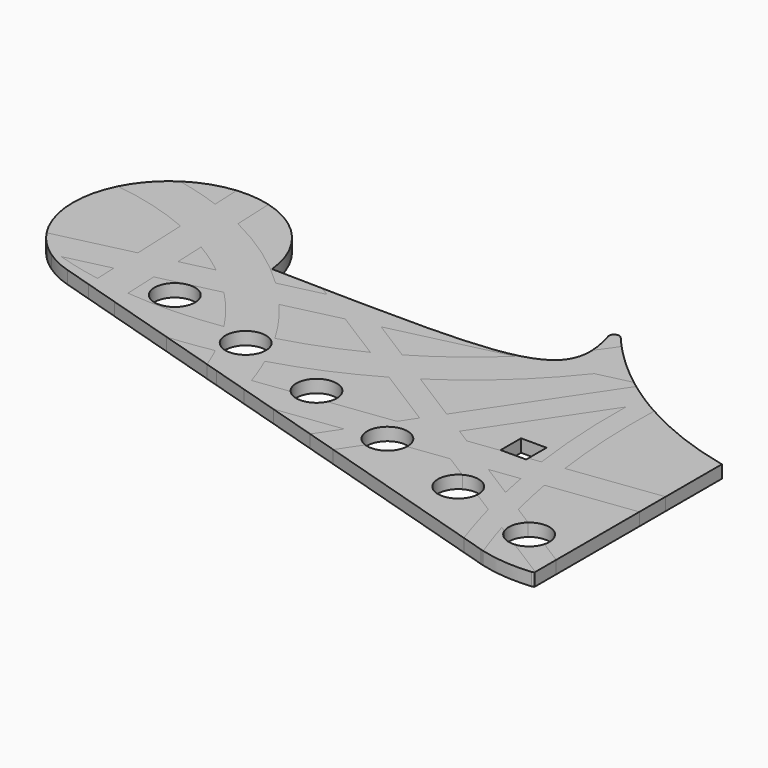
from build123d import *

# Parameters (mm, degrees)
F2_DEPTH    = 3.175
F3_DEPTH    = 3.175
F4_DEPTH    = 3.175
F5_R        = 5.0419
F6_DEPTH    = 3.1760001
F7_T1_DEPTH = 45.676518948
F8_W        = 6.35
F8_H        = 6.35
F9_DEPTH    = 25.4


# Not quite as in the source:
# - a fillet or chamfer that OpenCascade refuses, or shapes differently, is made with other operations: its cross-section is extruded or revolved along the edge and cut away or added
# - a feature names something its author has since deleted; it is built from what else it names


with BuildPart() as f2:
    # F1 (on Top) → F2 (new body)
    with BuildSketch(Plane.XY):
        with BuildLine():
            ThreePointArc((42.4964314187, 15.2975389884), (41.0489158835, 16.1252283316), (39.6171787622, 16.9799210768))
            Line((39.6171787622, 16.9799210768), (37.1046395912, 13.2316301906))
            ThreePointArc((37.1046395912, 13.2316301906), (37.366013418, -0.9466040935), (38.7394922855, -15.0605758765))
            Line((38.7394922855, -15.0605758765), (44.0297445972, -14.3774880883))
            ThreePointArc((44.0297445972, -14.3774880883), (42.6327723421, 0.4274569434), (42.4964314187, 15.2975389884))
        make_face()
        with BuildLine():
            Line((37.1046395912, 13.2316301906), (39.6171787622, 16.9799210768))
            ThreePointArc((39.6171787622, 16.9799210768), (38.4473968067, 17.7056848073), (37.2889933653, 18.4494752905))
            ThreePointArc((37.2889933653, 18.4494752905), (37.1779511751, 15.8412192781), (37.1046395912, 13.2316301906))
        make_face()
        with BuildLine():
            Line((18.2347737019, -14.9190737474), (37.1046395912, 13.2316301906))
            ThreePointArc((37.1046395912, 13.2316301906), (37.1779511751, 15.8412192781), (37.2889933653, 18.4494752905))
            ThreePointArc((37.2889933653, 18.4494752905), (35.2714811063, 19.8067738157), (33.291844794, 21.2187423255))
            Line((33.291844794, 21.2187423255), (11.7897327142, -10.8588354777))
            Line((11.7897327142, -10.8588354777), (18.2347737019, -14.9190737474))
        make_face()
        Polygon((21.909005611, -17.2337614333), (18.2347737019, -14.9190737474), (16.1880374428, -17.9724641003), align=None)
        Polygon((16.1880374428, -17.9724641003), (18.2347737019, -14.9190737474), (11.7897327142, -10.8588354777), (8.7250037822, -15.4309017191), (13.3425786538, -18.3398753382), align=None)
        with BuildLine():
            ThreePointArc((40.0179483598, -23.0484418301), (39.3339699918, -19.0616711332), (38.7394922855, -15.0605758765))
            Line((38.7394922855, -15.0605758765), (21.909005611, -17.2337614333))
            Line((21.909005611, -17.2337614333), (32.6492717175, -23.9998998575))
            Line((32.6492717175, -23.9998998575), (40.0179483598, -23.04844183))
        make_face()
        with BuildLine():
            Line((44.0297445972, -14.3774880883), (38.7394922855, -15.0605758765))
            ThreePointArc((38.7394922855, -15.0605758765), (39.3339699918, -19.0616711332), (40.0179483598, -23.0484418301))
            Line((40.0179483598, -23.04844183), (45.3156103763, -22.3643972862))
            ThreePointArc((45.3156103763, -22.3643972862), (44.6265684594, -18.3783660871), (44.0297445972, -14.3774880883))
        make_face()
        with BuildLine():
            Line((66.0969165157, -11.5281314286), (44.0297445972, -14.3774880883))
            ThreePointArc((44.0297445972, -14.3774880883), (44.6265684594, -18.3783660871), (45.3156103763, -22.3643972862))
            Line((45.3156103763, -22.3643972862), (66.0969165157, -19.6810741461))
            Line((66.0969165157, -19.6810741461), (66.0969165157, -11.5281314286))
        make_face()
        Polygon((21.909005611, -17.2337614333), (16.1880374428, -17.9724641003), (15.1700447699, -19.4911399889), (24.0828447602, -25.1060137624), (32.6492717175, -23.9998998575), align=None)
        Polygon((15.1700447699, -19.4911399889), (16.1880374428, -17.9724641003), (13.3425786538, -18.3398753382), align=None)
        with BuildLine():
            Line((8.7250037822, -15.4309017191), (11.7897327142, -10.8588354777))
            Line((11.7897327142, -10.8588354777), (-1.4386667359, -2.5252261497))
            ThreePointArc((-1.4386667359, -2.5252261497), (-4.0267817378, -4.16929298), (-6.661363794, -5.7378185279))
            Line((-6.661363794, -5.7378185279), (8.7250037822, -15.4309017191))
        make_face()
        with BuildLine():
            Line((45.3156103763, -22.3643972862), (40.0179483598, -23.04844183))
            ThreePointArc((40.0179483598, -23.0484418301), (40.6358918873, -26.2586545513), (41.3118678172, -29.4571505199))
            Line((41.3118678172, -29.4571505199), (47.7543417747, -33.5157716153))
            ThreePointArc((47.7543417747, -33.5157716153), (46.4441248758, -27.9599530039), (45.3156103763, -22.3643972862))
        make_face()
        with BuildLine():
            Line((23.5653367152, 20.3479618092), (31.8543854329, 22.2964799735))
            ThreePointArc((31.8543854329, 22.2964799735), (29.6938437842, 24.004445014), (27.5872449715, 25.7785155417))
            ThreePointArc((27.5872449715, 25.7785155417), (25.6195765344, 23.0311809725), (23.5653367152, 20.3479618092))
        make_face()
        Polygon((66.7319165157, -11.4461389791), (66.0969165157, -11.5281314286), (66.0969165157, -19.6810741461), (66.7319165157, -19.5990816966), align=None)
        Polygon((24.0828447602, -25.1060137624), (15.1700447699, -19.4911399889), (10.2051564991, -26.8979281778), align=None)
        Polygon((10.2051564991, -26.8979281778), (15.1700447699, -19.4911399889), (13.3425786538, -18.3398753382), (6.1527769462, -19.2682366821), (0.1698960025, -28.1937007596), align=None)
        Polygon((6.1527769462, -19.2682366821), (13.3425786538, -18.3398753382), (8.7250037822, -15.4309017191), align=None)
        with BuildLine():
            ThreePointArc((-6.661363794, -5.7378185279), (-4.0267817378, -4.16929298), (-1.4386667359, -2.5252261497))
            Line((-1.4386667359, -2.5252261497), (-10.5116171088, 3.1905389469))
            ThreePointArc((-10.5116171088, 3.1905389469), (-13.2464904723, 1.6325505109), (-16.0307927047, 0.16472172))
            Line((-16.0307927047, 0.16472172), (-6.661363794, -5.7378185279))
        make_face()
        with BuildLine():
            Line((-10.5116171088, 3.1905389469), (-1.4386667359, -2.5252261497))
            ThreePointArc((-1.4386667359, -2.5252261497), (11.983278832, 7.905724058), (23.5653367152, 20.3479618092))
            Line((23.5653367152, 20.3479618092), (6.9924854196, 16.4521586978))
            ThreePointArc((6.9924854196, 16.4521586978), (-1.3805057538, 9.3210248182), (-10.5116171088, 3.1905389469))
        make_face()
        with BuildLine():
            Line((41.3118678172, -29.4571505199), (32.6492717175, -23.9998998575))
            Line((32.6492717175, -23.9998998575), (24.0828447602, -25.1060137624))
            Line((24.0828447602, -25.1060137624), (43.1859281666, -37.140548603))
            ThreePointArc((43.1859281666, -37.140548603), (42.2068160775, -33.3091137761), (41.3118678172, -29.4571505199))
        make_face()
        with BuildLine():
            Line((47.7543417747, -33.5157716153), (41.3118678172, -29.4571505199))
            ThreePointArc((41.3118678172, -29.4571505199), (42.2068160775, -33.3091137761), (43.1859281666, -37.140548603))
            Line((43.1859281666, -37.140548603), (49.9469070818, -41.3998210243))
            ThreePointArc((49.9469070818, -41.3998210243), (48.8045830594, -37.4706004897), (47.7543417747, -33.5157716153))
        make_face()
        with BuildLine():
            Line((6.9924854196, 16.4521586978), (23.5653367152, 20.3479618092))
            ThreePointArc((23.5653367152, 20.3479618092), (25.6195765344, 23.0311809725), (27.5872449715, 25.7785155417))
            ThreePointArc((27.5872449715, 25.7785155417), (26.020865796, 27.172423594), (24.4877966317, 28.6028858679))
            Line((24.4877966317, 28.6028858679), (17.1245144057, 26.8719889151))
            add(Edge.make_bspline(
                [(7.6808851652, 17.1163986448), (14.1067211356, 18.8048631178), (17.0282926135, 21.7855138574), (17.1245144057, 26.8719889151)],
                knots=[0.4777006236, 0.4777006236, 0.4777006236, 0.4777006236, 0.7763446793, 0.7763446793, 0.7763446793, 0.7763446793], degree=3))
            ThreePointArc((7.6808851652, 17.1163986448), (7.3375096508, 16.7834243292), (6.9924854196, 16.4521586978))
        make_face()
        with BuildLine():
            Line((66.0969165157, -45.0712022279), (47.7543417747, -33.5157716153))
            ThreePointArc((47.7543417747, -33.5157716153), (48.8045830594, -37.4706004897), (49.9469070818, -41.3998210243))
            Line((49.9469070818, -41.3998210243), (66.0969165157, -51.5739822879))
            Line((66.0969165157, -51.5739822879), (66.0969165157, -45.0712022279))
        make_face()
        with BuildLine():
            Line((17.1245144057, 26.8719889151), (24.4877966317, 28.6028858679))
            ThreePointArc((24.4877966317, 28.6028858679), (22.4906185602, 30.5721371514), (20.5565558022, 32.6034106718))
            ThreePointArc((20.5565558022, 32.6034106718), (18.8719024579, 30.1633774038), (17.1129665679, 27.7763366052))
            add(Edge.make_bspline(
                [(17.1245144057, 26.8719889151), (17.1300825818, 27.1663337688), (17.1261894483, 27.4677304421), (17.1129665679, 27.7763366052)],
                knots=[0.7763446793, 0.7763446793, 0.7763446793, 0.7763446793, 0.7936266555, 0.7936266555, 0.7936266555, 0.7936266555], degree=3))
        make_face()
        Polygon((3.9051852235, -36.2964383336), (10.2051564991, -26.8979281778), (0.1698960025, -28.1937007596), (-3.7024240646, -33.9705587617), align=None)
        with BuildLine():
            Line((0.1698960025, -28.1937007596), (6.1527769462, -19.2682366821))
            Line((6.1527769462, -19.2682366821), (-26.6654353374, -23.5057888287))
            ThreePointArc((-26.6654353374, -23.5057888287), (-26.0722508431, -25.3958668205), (-25.5232745108, -27.2992552847))
            Line((-25.5232745108, -27.2992552847), (-15.8372389855, -30.2605735265))
            Line((-15.8372389855, -30.2605735265), (0.1698960025, -28.1937007596))
        make_face()
        with BuildLine():
            ThreePointArc((-29.6968030266, -15.588280186), (-17.887048807, -11.3459762685), (-6.661363794, -5.7378185279))
            Line((-6.661363794, -5.7378185279), (-16.0307927047, 0.16472172))
            ThreePointArc((-16.0307927047, 0.16472172), (-24.9308801058, -3.7912137914), (-34.1848701937, -6.8284245133))
            ThreePointArc((-34.1848701937, -6.8284245133), (-31.813933797, -11.1433343436), (-29.6968030266, -15.588280186))
        make_face()
        with BuildLine():
            ThreePointArc((-16.0307927047, 0.16472172), (-13.2464904723, 1.6325505109), (-10.5116171088, 3.1905389469))
            Line((-10.5116171088, 3.1905389469), (-21.0854633248, 9.8518363918))
            Line((-21.0854633248, 9.8518363918), (-28.6026932396, 8.0847507426))
            Line((-28.6026932396, 8.0847507426), (-16.0307927047, 0.16472172))
        make_face()
        with BuildLine():
            Line((49.9469070818, -41.3998210243), (43.1859281666, -37.140548603))
            ThreePointArc((43.1859281666, -37.140548603), (44.9597148144, -43.3326667725), (46.9532808608, -49.4575619483))
            Line((46.9532808608, -49.4575619483), (52.654517861, -51.2006050215))
            add(Edge.make_bspline(
                [(52.654517861, -51.2006050215), (52.8721432701, -51.2671397861), (53.0908731316, -51.3311050786), (53.3106253892, -51.392535085)],
                knots=[0, 0, 0, 0, 0.0179188265, 0.0179188265, 0.0179188265, 0.0179188265], degree=3))
            ThreePointArc((53.3106253892, -51.392535085), (51.5535715097, -46.4214898843), (49.9469070818, -41.3998210243))
        make_face()
        with BuildLine():
            Line((-21.0854633248, 9.8518363918), (6.9924854196, 16.4521586978))
            ThreePointArc((6.9924854196, 16.4521586978), (7.3375096508, 16.7834243292), (7.6808851652, 17.1163986448))
            add(Edge.make_bspline(
                [(-29.5465874229, 15.1821639931), (-11.7884739785, 14.9407807553), (0.2741126095, 15.1701814713), (7.6808851652, 17.1163986448)],
                knots=[0.1334670318, 0.1334670318, 0.1334670318, 0.1334670318, 0.4777006236, 0.4777006236, 0.4777006236, 0.4777006236], degree=3))
            Line((-29.5465874229, 15.1821639931), (-21.0854633248, 9.8518363918))
        make_face()
        Polygon((66.7319165157, -45.4712386755), (66.0969165157, -45.0712022279), (66.0969165157, -51.5739822879), (66.7319165157, -51.9740187355), (66.7319165157, -50.6766184161), align=None)
        with BuildLine():
            ThreePointArc((-25.5232745108, -27.2992552847), (-26.0722508431, -25.3958668205), (-26.6654353374, -23.5057888287))
            Line((-26.6654353374, -23.5057888287), (-34.5859869423, -24.5285060372))
            Line((-34.5859869423, -24.5285060372), (-25.5232745108, -27.2992552847))
        make_face()
        with BuildLine():
            Line((-34.5859869423, -24.5285060372), (-26.6654353374, -23.5057888287))
            ThreePointArc((-26.6654353374, -23.5057888287), (-28.082343762, -19.5092164726), (-29.6968030266, -15.588280186))
            ThreePointArc((-29.6968030266, -15.588280186), (-34.8240491393, -16.9555811432), (-40.0132953676, -18.0645843849))
            ThreePointArc((-40.0132953676, -18.0645843849), (-38.7883325091, -20.8009357195), (-37.6743280791, -23.5843053969))
            Line((-37.6743280791, -23.5843053969), (-34.5859869423, -24.5285060372))
        make_face()
        with BuildLine():
            ThreePointArc((-40.0132953676, -18.0645843849), (-34.8240491393, -16.9555811432), (-29.6968030266, -15.588280186))
            ThreePointArc((-29.6968030266, -15.588280186), (-31.813933797, -11.1433343436), (-34.1848701937, -6.8284245133))
            ThreePointArc((-34.1848701937, -6.8284245133), (-39.5644417055, -8.1325608515), (-45.0100273339, -9.1256159374))
            ThreePointArc((-45.0100273339, -9.1256159374), (-42.3580614142, -13.5092403981), (-40.0132953676, -18.0645843849))
        make_face()
        with BuildLine():
            Line((-28.6026932396, 8.0847507426), (-21.0854633248, 9.8518363918))
            Line((-21.0854633248, 9.8518363918), (-29.5465874229, 15.1821639931))
            add(Edge.make_bspline(
                [(-32.4245408212, 15.2244238657), (-31.4490517341, 15.209133599), (-30.4897858638, 15.1949847409), (-29.5465874229, 15.1821639931)],
                knots=[0.1151835251, 0.1151835251, 0.1151835251, 0.1151835251, 0.1334670318, 0.1334670318, 0.1334670318, 0.1334670318], degree=3))
            Line((-32.4245408212, 15.2244238657), (-37.8947338501, 13.9385380129))
            Line((-37.8947338501, 13.9385380129), (-28.6026932396, 8.0847507426))
        make_face()
        with BuildLine():
            Line((-42.4321868943, 4.8338325121), (-28.6026932396, 8.0847507426))
            Line((-28.6026932396, 8.0847507426), (-37.8947338501, 13.9385380129))
            Line((-37.8947338501, 13.9385380129), (-48.6032420976, 11.4212741454))
            ThreePointArc((-48.6032420976, 11.4212741454), (-45.430208748, 8.2095279148), (-42.4321868943, 4.8338325121))
        make_face()
        with BuildLine():
            ThreePointArc((-45.0100273339, -9.1256159374), (-39.5644417055, -8.1325608515), (-34.1848701937, -6.8284245133))
            ThreePointArc((-34.1848701937, -6.8284245133), (-38.0631186166, -0.8237469707), (-42.4321868943, 4.8338325121))
            Line((-42.4321868943, 4.8338325121), (-54.0070813026, 2.1129060495))
            ThreePointArc((-54.0070813026, 2.1129060495), (-49.23676466, -3.2887723983), (-45.0100273339, -9.1256159374))
        make_face()
        with BuildLine():
            ThreePointArc((-50.9314824477, -19.5311865576), (-45.4533242171, -18.9398134331), (-40.0132953676, -18.0645843849))
            ThreePointArc((-40.0132953676, -18.0645843849), (-42.3580614142, -13.5092403981), (-45.0100273339, -9.1256159374))
            ThreePointArc((-45.0100273339, -9.1256159374), (-56.6586871971, -10.1875434452), (-68.3501889524, -9.8301174407))
            Line((-68.3501889524, -9.8301174407), (-68.1593155628, -14.2641093992))
            Line((-68.1593155628, -14.2641093992), (-50.9314824477, -19.5311865576))
        make_face()
        with BuildLine():
            Line((-40.1503334653, 15.3595176307), (-37.8947338501, 13.9385380129))
            Line((-37.8947338501, 13.9385380129), (-32.4245408212, 15.2244238657))
            add(Edge.make_bspline(
                [(-40.1503334653, 15.3595176307), (-37.4693381201, 15.3091877057), (-34.8949173044, 15.2631456884), (-32.4245408212, 15.2244238657)],
                knots=[0.0688814745, 0.0688814745, 0.0688814745, 0.0688814745, 0.1151835251, 0.1151835251, 0.1151835251, 0.1151835251], degree=3))
        make_face()
        with BuildLine():
            Line((-54.0070813026, 2.1129060495), (-42.4321868943, 4.8338325121))
            ThreePointArc((-42.4321868943, 4.8338325121), (-45.430208748, 8.2095279148), (-48.6032420976, 11.4212741454))
            Line((-48.6032420976, 11.4212741454), (-61.0611600505, 8.492774115))
            ThreePointArc((-61.0611600505, 8.492774115), (-57.4323204183, 5.4153983721), (-54.0070813026, 2.1129060495))
        make_face()
        with BuildLine():
            Line((-61.0611600505, 8.492774115), (-48.6032420976, 11.4212741454))
            ThreePointArc((-48.6032420976, 11.4212741454), (-58.6808959079, 19.7062783812), (-69.9077254027, 26.3514797328))
            Line((-69.9077254027, 26.3514797328), (-69.3860241765, 14.2323517303))
            ThreePointArc((-69.3860241765, 14.2323517303), (-65.1262135584, 11.5038038457), (-61.0611600505, 8.492774115))
        make_face()
        with BuildLine():
            Line((-68.7154707451, -1.3446154313), (-54.0070813026, 2.1129060495))
            ThreePointArc((-54.0070813026, 2.1129060495), (-57.4323204183, 5.4153983721), (-61.0611600505, 8.492774115))
            Line((-61.0611600505, 8.492774115), (-69.0580256175, 6.6129398486))
            Line((-69.0580256175, 6.6129398486), (-68.7154707451, -1.3446154313))
        make_face()
        with BuildLine():
            ThreePointArc((-76.8586239766, -8.6668452954), (-72.6173728923, -9.3433207475), (-68.3501889524, -9.8301174407))
            Line((-68.3501889524, -9.8301174407), (-68.7154707451, -1.3446154313))
            Line((-68.7154707451, -1.3446154313), (-77.0890943511, -3.3130147318))
            Line((-77.0890943511, -3.3130147318), (-76.8586239766, -8.6668452954))
        make_face()
        with BuildLine():
            Line((-68.1593155628, -14.2641093992), (-68.3501889524, -9.8301174407))
            ThreePointArc((-68.3501889524, -9.8301174407), (-72.6173728923, -9.3433207475), (-76.8586239766, -8.6668452954))
            Line((-76.8586239766, -8.6668452954), (-76.730479586, -11.6436415815))
            Line((-76.730479586, -11.6436415815), (-68.1593155628, -14.2641093992))
        make_face()
        with BuildLine():
            ThreePointArc((-78.5240021741, 30.0199174278), (-74.1653042963, 28.3044506523), (-69.9077254027, 26.3514797328))
            Line((-69.9077254027, 26.3514797328), (-70.3394310892, 36.3800098813))
            ThreePointArc((-70.3394310892, 36.3800098813), (-74.5513100111, 37.131060612), (-78.829611199, 37.1192200675))
            Line((-78.829611199, 37.1192200675), (-78.5240021741, 30.0199174278))
        make_face()
        with BuildLine():
            Line((-69.3860241765, 14.2323517303), (-69.9077254027, 26.3514797328))
            ThreePointArc((-69.9077254027, 26.3514797328), (-74.1653042963, 28.3044506523), (-78.5240021741, 30.0199174278))
            Line((-78.5240021741, 30.0199174278), (-78.0338005415, 18.6325254977))
            ThreePointArc((-78.0338005415, 18.6325254977), (-73.6382831604, 16.5732133478), (-69.3860241765, 14.2323517303))
        make_face()
        Polygon((-77.0890943511, -3.3130147318), (-68.7154707451, -1.3446154313), (-69.0580256175, 6.6129398486), (-77.4316492235, 4.6445405481), align=None)
        with BuildLine():
            Line((-76.730479586, -11.6436415815), (-76.8586239766, -8.6668452954))
            ThreePointArc((-76.8586239766, -8.6668452954), (-82.5281158651, -7.4551998292), (-88.1144721554, -5.904765565))
            Line((-88.1144721554, -5.904765565), (-90.1562794913, -6.3847360439))
            ThreePointArc((-90.1562794913, -6.3847360439), (-87.0051766902, -8.2121096218), (-83.6129915736, -9.5394465014))
            Line((-83.6129915736, -9.5394465014), (-76.730479586, -11.6436415815))
        make_face()
        with BuildLine():
            Line((-77.4316492235, 4.6445405481), (-69.0580256175, 6.6129398486))
            Line((-69.0580256175, 6.6129398486), (-69.3860241765, 14.2323517303))
            ThreePointArc((-69.3860241765, 14.2323517303), (-73.6382831604, 16.5732133478), (-78.0338005415, 18.6325254977))
            Line((-78.0338005415, 18.6325254977), (-77.4316492235, 4.6445405481))
        make_face()
        with BuildLine():
            Line((-78.0338005415, 18.6325254977), (-78.5240021741, 30.0199174278))
            ThreePointArc((-78.5240021741, 30.0199174278), (-84.1174389484, 31.8289833917), (-89.8225422612, 33.2470986199))
            ThreePointArc((-89.8225422612, 33.2470986199), (-94.4940594414, 29.1935052495), (-97.9690847289, 24.0769740779))
            ThreePointArc((-97.9690847289, 24.0769740779), (-87.8119657312, 22.0485346354), (-78.0338005415, 18.6325254977))
        make_face()
        with BuildLine():
            Line((-88.1144721554, -5.904765565), (-77.0890943511, -3.3130147318))
            Line((-77.0890943511, -3.3130147318), (-77.4316492235, 4.6445405481))
            Line((-77.4316492235, 4.6445405481), (-96.5696239893, 0.1457503093))
            ThreePointArc((-96.5696239893, 0.1457503093), (-94.7885596821, -2.218402202), (-92.7289486745, -4.3442925239))
            ThreePointArc((-92.7289486745, -4.3442925239), (-90.4315734951, -5.1536951694), (-88.1144721554, -5.904765565))
        make_face()
        with BuildLine():
            Line((-90.1562794913, -6.3847360439), (-88.1144721554, -5.904765565))
            ThreePointArc((-88.1144721554, -5.904765565), (-90.4315734951, -5.1536951694), (-92.7289486745, -4.3442925239))
            ThreePointArc((-92.7289486745, -4.3442925239), (-91.4776936841, -5.408743986), (-90.1562794913, -6.3847360439))
        make_face()
    extrude(amount=F2_DEPTH)


with BuildPart() as f3:
    # F1 (on Top) → F3 (new body)
    with BuildSketch(Plane.XY):
        with BuildLine():
            Line((66.0969165157, -19.6810741461), (45.3156103763, -22.3643972862))
            ThreePointArc((45.3156103763, -22.3643972862), (46.4441248758, -27.9599530039), (47.7543417747, -33.5157716153))
            Line((47.7543417747, -33.5157716153), (66.0969165157, -45.0712022279))
            Line((66.0969165157, -45.0712022279), (66.0969165157, -19.6810741461))
        make_face()
        Polygon((66.7319165157, -19.5990816966), (66.0969165157, -19.6810741461), (66.0969165157, -45.0712022279), (66.7319165157, -45.4712386755), align=None)
    extrude(amount=F3_DEPTH)


with BuildPart() as f3b:
    # F1 (on Top) → F3, piece 2 (new body)
    with BuildSketch(Plane.XY):
        with BuildLine():
            ThreePointArc((38.7394922855, -15.0605758765), (37.366013418, -0.9466040935), (37.1046395912, 13.2316301906))
            Line((37.1046395912, 13.2316301906), (18.2347737019, -14.9190737474))
            Line((18.2347737019, -14.9190737474), (21.909005611, -17.2337614333))
            Line((21.909005611, -17.2337614333), (38.7394922855, -15.0605758765))
        make_face()
    extrude(amount=F3_DEPTH)


with BuildPart() as f3c:
    # F1 (on Top) → F3, piece 3 (new body)
    with BuildSketch(Plane.XY):
        with BuildLine():
            ThreePointArc((41.3118678172, -29.4571505199), (40.6358918873, -26.2586545513), (40.0179483598, -23.0484418301))
            Line((40.0179483598, -23.04844183), (32.6492717175, -23.9998998575))
            Line((32.6492717175, -23.9998998575), (41.3118678172, -29.4571505199))
        make_face()
    extrude(amount=F3_DEPTH)


with BuildPart() as f3d:
    # F1 (on Top) → F3, piece 4 (new body)
    with BuildSketch(Plane.XY):
        with BuildLine():
            Line((24.0828447602, -25.1060137624), (10.2051564991, -26.8979281778))
            Line((10.2051564991, -26.8979281778), (3.9051852235, -36.2964383336))
            Line((3.9051852235, -36.2964383336), (46.9532808608, -49.4575619483))
            ThreePointArc((46.9532808608, -49.4575619483), (44.9597148144, -43.3326667725), (43.1859281666, -37.140548603))
            Line((43.1859281666, -37.140548603), (24.0828447602, -25.1060137624))
        make_face()
    extrude(amount=F3_DEPTH)


with BuildPart() as f3e:
    # F1 (on Top) → F3, piece 5 (new body)
    with BuildSketch(Plane.XY):
        with BuildLine():
            Line((66.0969165157, -51.5739822879), (49.9469070818, -41.3998210243))
            ThreePointArc((49.9469070818, -41.3998210243), (51.5535715097, -46.4214898843), (53.3106253892, -51.392535085))
            add(Edge.make_bspline(
                [(53.3106253892, -51.392535085), (57.3951470823, -52.5343308356), (61.832880342, -52.8002504688), (66.0969165157, -52.4098137845)],
                knots=[0.0179188265, 0.0179188265, 0.0179188265, 0.0179188265, 0.3509749519, 0.3509749519, 0.3509749519, 0.3509749519], degree=3))
            Line((66.0969165157, -52.4098137845), (66.0969165157, -51.5739822879))
        make_face()
        with BuildLine():
            Line((66.7319165157, -51.9740187355), (66.0969165157, -51.5739822879))
            Line((66.0969165157, -51.5739822879), (66.0969165157, -52.4098137845))
            ThreePointArc((66.0969165157, -52.4098137845), (66.426687168, -52.3406803211), (66.7319165157, -52.1979807617))
            Line((66.7319165157, -52.1979807617), (66.7319165157, -51.9740187355))
        make_face()
    extrude(amount=F3_DEPTH)


with BuildPart() as f3f:
    # F1 (on Top) → F3, piece 6 (new body)
    with BuildSketch(Plane.XY):
        with BuildLine():
            ThreePointArc((66.0969165157, 6.2159453417), (53.9721180988, 9.9133135519), (42.4964314187, 15.2975389884))
            ThreePointArc((42.4964314187, 15.2975389884), (42.6327723421, 0.4274569434), (44.0297445972, -14.3774880883))
            Line((44.0297445972, -14.3774880883), (66.0969165157, -11.5281314286))
            Line((66.0969165157, -11.5281314286), (66.0969165157, 6.2159453417))
        make_face()
        with BuildLine():
            ThreePointArc((66.7319165157, 6.0732997692), (66.4142859791, 6.1440414601), (66.0969165157, 6.2159453417))
            Line((66.0969165157, 6.2159453417), (66.0969165157, -11.5281314286))
            Line((66.0969165157, -11.5281314286), (66.7319165157, -11.4461389791))
            Line((66.7319165157, -11.4461389791), (66.7319165157, 6.0732997692))
        make_face()
    extrude(amount=F3_DEPTH)


with BuildPart() as f4:
    # F1 (on Top) → F4 (new body)
    with BuildSketch(Plane.XY):
        with BuildLine():
            Line((-69.0580256175, 6.6129398486), (-61.0611600505, 8.492774115))
            ThreePointArc((-61.0611600505, 8.492774115), (-65.1262135584, 11.5038038457), (-69.3860241765, 14.2323517303))
            Line((-69.3860241765, 14.2323517303), (-69.0580256175, 6.6129398486))
        make_face()
    extrude(amount=F4_DEPTH)


with BuildPart() as f4b:
    # F1 (on Top) → F4, piece 2 (new body)
    with BuildSketch(Plane.XY):
        with BuildLine():
            Line((-96.5696239893, 0.1457503093), (-77.4316492235, 4.6445405481))
            Line((-77.4316492235, 4.6445405481), (-78.0338005415, 18.6325254977))
            ThreePointArc((-78.0338005415, 18.6325254977), (-87.8119657312, 22.0485346354), (-97.9690847289, 24.0769740779))
            ThreePointArc((-97.9690847289, 24.0769740779), (-100.4863179642, 11.9232391662), (-96.5696239893, 0.1457503093))
        make_face()
    extrude(amount=F4_DEPTH)


with BuildPart() as f4c:
    # F1 (on Top) → F4, piece 3 (new body)
    with BuildSketch(Plane.XY):
        with BuildLine():
            ThreePointArc((-89.8225422612, 33.2470986199), (-84.1174389484, 31.8289833917), (-78.5240021741, 30.0199174278))
            Line((-78.5240021741, 30.0199174278), (-78.829611199, 37.1192200675))
            ThreePointArc((-78.829611199, 37.1192200675), (-84.5656995824, 35.8634472767), (-89.8225422612, 33.2470986199))
        make_face()
    extrude(amount=F4_DEPTH)


with BuildPart() as f4d:
    # F1 (on Top) → F4, piece 4 (new body)
    with BuildSketch(Plane.XY):
        with BuildLine():
            ThreePointArc((-68.3501889524, -9.8301174407), (-56.6586871971, -10.1875434452), (-45.0100273339, -9.1256159374))
            ThreePointArc((-45.0100273339, -9.1256159374), (-49.23676466, -3.2887723983), (-54.0070813026, 2.1129060495))
            Line((-54.0070813026, 2.1129060495), (-68.7154707451, -1.3446154313))
            Line((-68.7154707451, -1.3446154313), (-68.3501889524, -9.8301174407))
        make_face()
    extrude(amount=F4_DEPTH)


with BuildPart() as f4e:
    # F1 (on Top) → F4, piece 5 (new body)
    with BuildSketch(Plane.XY):
        with BuildLine():
            ThreePointArc((-34.1848701937, -6.8284245133), (-24.9308801058, -3.7912137914), (-16.0307927047, 0.16472172))
            Line((-16.0307927047, 0.16472172), (-28.6026932396, 8.0847507426))
            Line((-28.6026932396, 8.0847507426), (-42.4321868943, 4.8338325121))
            ThreePointArc((-42.4321868943, 4.8338325121), (-38.0631186166, -0.8237469707), (-34.1848701937, -6.8284245133))
        make_face()
    extrude(amount=F4_DEPTH)


with BuildPart() as f4f:
    # F1 (on Top) → F4, piece 6 (new body)
    with BuildSketch(Plane.XY):
        with BuildLine():
            Line((6.1527769462, -19.2682366821), (8.7250037822, -15.4309017191))
            Line((8.7250037822, -15.4309017191), (-6.661363794, -5.7378185279))
            ThreePointArc((-6.661363794, -5.7378185279), (-17.887048807, -11.3459762685), (-29.6968030266, -15.588280186))
            ThreePointArc((-29.6968030266, -15.588280186), (-28.082343762, -19.5092164726), (-26.6654353374, -23.5057888287))
            Line((-26.6654353374, -23.5057888287), (6.1527769462, -19.2682366821))
        make_face()
    extrude(amount=F4_DEPTH)


with BuildPart() as f4g:
    # F1 (on Top) → F4, piece 7 (new body)
    with BuildSketch(Plane.XY):
        Polygon((-3.7024240646, -33.9705587617), (0.1698960025, -28.1937007596), (-15.8372389855, -30.2605735265), align=None)
    extrude(amount=F4_DEPTH)


with BuildPart() as f4h:
    # F1 (on Top) → F4, piece 8 (new body)
    with BuildSketch(Plane.XY):
        with BuildLine():
            Line((11.7897327142, -10.8588354777), (33.291844794, 21.2187423255))
            ThreePointArc((33.291844794, 21.2187423255), (32.5703924984, 21.7539797942), (31.8543854329, 22.2964799735))
            Line((31.8543854329, 22.2964799735), (23.5653367152, 20.3479618092))
            ThreePointArc((23.5653367152, 20.3479618092), (11.983278832, 7.905724058), (-1.4386667359, -2.5252261497))
            Line((-1.4386667359, -2.5252261497), (11.7897327142, -10.8588354777))
        make_face()
    extrude(amount=F4_DEPTH)


with BuildPart() as f4i:
    # F1 (on Top) → F4, piece 9 (new body)
    with BuildSketch(Plane.XY):
        with BuildLine():
            Line((-48.6032420976, 11.4212741454), (-37.8947338501, 13.9385380129))
            Line((-37.8947338501, 13.9385380129), (-40.1503334653, 15.3595176307))
            add(Edge.make_bspline(
                [(-52.8314374799, 15.6026238776), (-48.3629873437, 15.5187543961), (-44.1387294409, 15.4343911923), (-40.1503334653, 15.3595176307)],
                knots=[0, 0, 0, 0, 0.0688814745, 0.0688814745, 0.0688814745, 0.0688814745], degree=3))
            ThreePointArc((-52.8314374799, 15.6026238776), (-58.3461532671, 28.7208860054), (-70.3394310892, 36.3800098813))
            Line((-70.3394310892, 36.3800098813), (-69.9077254027, 26.3514797328))
            ThreePointArc((-69.9077254027, 26.3514797328), (-58.6808959079, 19.7062783812), (-48.6032420976, 11.4212741454))
        make_face()
    extrude(amount=F4_DEPTH)


with BuildPart() as f4j:
    # F1 (on Top) → F4, piece 10 (new body)
    with BuildSketch(Plane.XY):
        with BuildLine():
            Line((-21.0854633248, 9.8518363918), (-10.5116171088, 3.1905389469))
            ThreePointArc((-10.5116171088, 3.1905389469), (-1.3805057538, 9.3210248182), (6.9924854196, 16.4521586978))
            Line((6.9924854196, 16.4521586978), (-21.0854633248, 9.8518363918))
        make_face()
    extrude(amount=F4_DEPTH)


with BuildPart() as f4k:
    # F1 (on Top) → F4, piece 11 (new body)
    with BuildSketch(Plane.XY):
        with BuildLine():
            ThreePointArc((17.1129665679, 27.7763366052), (18.8719024579, 30.1633774038), (20.5565558022, 32.6034106718))
            ThreePointArc((20.5565558022, 32.6034106718), (16.5486237409, 37.2612109489), (12.8720226331, 42.1847490185))
            add(Edge.make_bspline(
                [(17.1129665679, 27.7763366052), (16.9550650635, 31.4615682759), (15.466738994, 36.1748752691), (12.8720226331, 42.1847490185)],
                knots=[0.7936266555, 0.7936266555, 0.7936266555, 0.7936266555, 1, 1, 1, 1], degree=3))
        make_face()
    extrude(amount=F4_DEPTH)

    # F7: fillet of radius 1.27 on 1 edges, made by hand

    # F7_s2 → F7_t1 (cut)
    with BuildSketch(Plane.XY.offset(-21.250759474)):
        with BuildLine():
            ThreePointArc((18.0481580543, 35.4421392407), (16.4710218075, 35.7371516836), (15.8625647413, 34.2525065809))
            Line((15.8625647413, 34.2525065809), (15.7409774272, 34.2156365615))
            ThreePointArc((15.7409774272, 34.2156365615), (14.3577735093, 38.214987165), (12.7553753574, 42.1343874623))
            Line((12.7553753574, 42.1343874623), (12.9763918727, 42.2572054544))
            ThreePointArc((12.9763918727, 42.2572054544), (15.4800803133, 38.8287884402), (18.1451300716, 35.5242324873))
            Line((18.1451300716, 35.5242324873), (18.0481580543, 35.4421392407))
        make_face()
    extrude(amount=F7_T1_DEPTH, mode=Mode.SUBTRACT)


with BuildPart() as f4l:
    # F1 (on Top) → F4, piece 12 (new body)
    with BuildSketch(Plane.XY):
        with BuildLine():
            ThreePointArc((-37.6743280791, -23.5843053969), (-38.7883325091, -20.8009357195), (-40.0132953676, -18.0645843849))
            ThreePointArc((-40.0132953676, -18.0645843849), (-45.4533242171, -18.9398134331), (-50.9314824477, -19.5311865576))
            Line((-50.9314824477, -19.5311865576), (-37.6743280791, -23.5843053969))
        make_face()
    extrude(amount=F4_DEPTH)


with BuildPart() as f4m:
    # F1 (on Top) → F4, piece 13 (new body)
    with BuildSketch(Plane.XY):
        with BuildLine():
            ThreePointArc((-88.1144721554, -5.904765565), (-82.5281158651, -7.4551998292), (-76.8586239766, -8.6668452954))
            Line((-76.8586239766, -8.6668452954), (-77.0890943511, -3.3130147318))
            Line((-77.0890943511, -3.3130147318), (-88.1144721554, -5.904765565))
        make_face()
    extrude(amount=F4_DEPTH)


with BuildPart() as f6_tool:
    # F5 (on Top) → F6 (new body, through all)
    with BuildSketch(Plane.XY):
        with Locations((-60.7603863453, -4.7372468837)):
            Circle(F5_R)
        with Locations((-37.4175610351, -11.873864773)):
            Circle(F5_R)
        with Locations((-14.0747357248, -19.0104826622)):
            Circle(F5_R)
        with Locations((9.2680895854, -26.1471005515)):
            Circle(F5_R)
        with Locations((32.6109148956, -33.2837184407)):
            Circle(F5_R)
        with Locations((55.9537402058, -40.42033633)):
            Circle(F5_R)
    extrude(amount=F6_DEPTH)


with BuildPart() as f2_1:
    add(f2.part)

    # F6: cut by f6_tool
    add(f6_tool.part, mode=Mode.SUBTRACT)


with BuildPart() as f3_1:
    add(f3.part)

    # F6: cut by f6_tool
    add(f6_tool.part, mode=Mode.SUBTRACT)


with BuildPart() as f3d_1:
    add(f3d.part)

    # F6: cut by f6_tool
    add(f6_tool.part, mode=Mode.SUBTRACT)


with BuildPart() as f3e_1:
    add(f3e.part)

    # F6: cut by f6_tool
    add(f6_tool.part, mode=Mode.SUBTRACT)


with BuildPart() as f4d_1:
    add(f4d.part)

    # F6: cut by f6_tool
    add(f6_tool.part, mode=Mode.SUBTRACT)


with BuildPart() as f4f_1:
    add(f4f.part)

    # F6: cut by f6_tool
    add(f6_tool.part, mode=Mode.SUBTRACT)


with BuildPart() as f9_tool:
    # F8 (on Top) → F9 (new body)
    with BuildSketch(Plane.XY):
        with Locations((32.6109148956, -12.9637184407)):
            Rectangle(F8_W, F8_H)
    extrude(amount=F9_DEPTH)


with BuildPart() as f2_2:
    add(f2_1.part)

    # F9: cut by f9_tool
    add(f9_tool.part, mode=Mode.SUBTRACT)


with BuildPart() as f3b_1:
    add(f3b.part)

    # F9: cut by f9_tool
    add(f9_tool.part, mode=Mode.SUBTRACT)


solid = Compound([f3c.part, f3f.part, f4.part, f4b.part, f4c.part, f4e.part, f4g.part, f4h.part, f4i.part, f4j.part, f4k.part, f4l.part, f4m.part, f3_1.part, f3d_1.part, f3e_1.part, f4d_1.part, f4f_1.part, f2_2.part, f3b_1.part])
